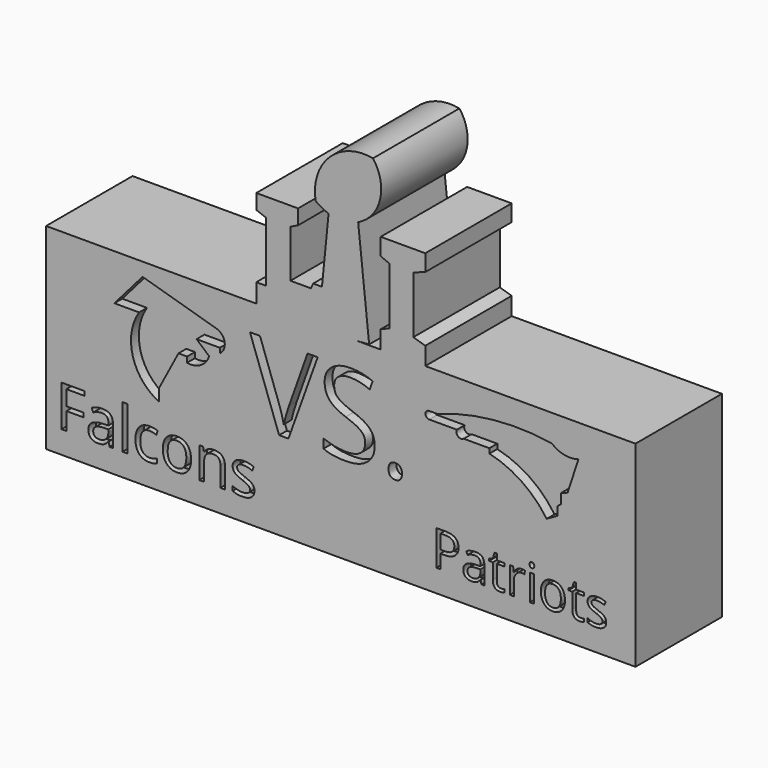
from build123d import *

# Parameters (mm, degrees)
F1_DEPTH       = 27.94
F2_TEXT_SIZE   = 14.8749987905
F2_TEXT_SIZE_2 = 12.6875005662
F2_TEXT_SIZE_3 = 29.4177713774
F3_DEPTH       = 2.54


# Not quite as in the source:
# - Text() gives the source's letters only with a copy of the font that has no kerning and outlines rounded to 1/6400 em; it was checked with that copy


with BuildPart() as f1:
    # F0 (on Front) → F1 (new body)
    with BuildSketch(Plane.XZ):
        Polygon((-20.7396647019, 6.5645907312), (-75.0956647019, 6.5645907312), (-75.0956647019, -44.2354092688), (77.3043352981, -44.2354092688), (77.3043352981, 6.5645907312), (22.9483352981, 6.5645907312), (11.4252582135, 6.5645907312), (5.2129668421, 6.5645907312), align=None)
        with BuildLine():
            Line((-20.7396647019, 11.4441978476), (-20.7396647019, 6.5645907312))
            Line((-20.7396647019, 6.5645907312), (5.2129668421, 6.5645907312))
            Line((5.2129668421, 6.5645907312), (3.6289432175, 32.9649871859))
            ThreePointArc((3.6289432175, 32.9649871859), (0.777301251, 32.6608543414), (-2.049780525, 33.1424842033))
            Line((-2.049780525, 33.1424842033), (-3.7631863539, 15.9227544818))
            Line((-3.7631863539, 15.9227544818), (-6.0277319506, 15.9227544818))
            Line((-6.0277319506, 15.9227544818), (-6.6274235949, 14.6377006922))
            Line((-6.6274235949, 14.6377006922), (-11.9156263826, 14.6377006922))
            Line((-11.9156263826, 14.6377006922), (-11.9156263826, 26.9505194119))
            Line((-11.9156263826, 26.9505194119), (-9.9452095164, 27.8928911975))
            Line((-9.9452095164, 27.8928911975), (-9.9452095164, 31.7480562917))
            Line((-9.9452095164, 31.7480562917), (-20.7396647019, 31.7480562917))
            Line((-20.7396647019, 31.7480562917), (-20.7396647019, 27.8928911975))
            Line((-20.7396647019, 27.8928911975), (-18.2552276237, 26.9505194119))
            Line((-18.2552276237, 26.9505194119), (-18.2552276237, 11.4441978476))
            Line((-18.2552276237, 11.4441978476), (-20.7396647019, 11.4441978476))
        make_face()
        with BuildLine():
            Line((3.6289432175, 32.9649871859), (5.2129668421, 6.5645907312))
            Line((5.2129668421, 6.5645907312), (8.4404846862, 6.758241782))
            Line((8.4404846862, 6.758241782), (5.5982306723, 33.6702211093))
            ThreePointArc((5.5982306723, 33.6702211093), (4.6312572936, 33.26826166), (3.6289432175, 32.9649871859))
        make_face()
        Polygon((11.4252582135, 11.1887202485), (11.4252582135, 6.5645907312), (22.9483352981, 6.5645907312), (22.9483352981, 11.1887202485), (19.8673630075, 12.1255040675), (19.8673630075, 26.8694617361), (22.9483352981, 27.9540222956), (22.9483352981, 32.2345261348), (11.4252582135, 32.2345261348), (11.4252582135, 27.8206810862), (13.6844111549, 26.8694617361), (13.6844111549, 12.1255040675), align=None)
        with BuildLine():
            ThreePointArc((-2.049780525, 33.1424842033), (0.777301251, 32.6608543414), (3.6289432175, 32.9649871859))
            ThreePointArc((3.6289432175, 32.9649871859), (4.6312572936, 33.26826166), (5.5982306723, 33.6702211093))
            ThreePointArc((5.5982306723, 33.6702211093), (11.2702064802, 40.6482895305), (9.43088028, 49.4506544164))
            ThreePointArc((9.43088028, 49.4506544164), (-1.7919494105, 46.0737788777), (-5.3994817717, 34.922953575))
            ThreePointArc((-5.3994817717, 34.922953575), (-3.8060075962, 33.8796206145), (-2.049780525, 33.1424842033))
        make_face()
    extrude(amount=F1_DEPTH)

    # F2 (on face) → F3 (cut)
    with BuildSketch(Plane.XZ.offset(27.94)):
        with BuildLine():
            Line((-57.4300996959, -5.2845505534), (-51.0407872498, -5.2845505534))
            ThreePointArc((-51.0407872498, -5.2845505534), (-52.6724909786, -15.8235590914), (-45.8401814103, -24.0121306388))
            Line((-45.8401814103, -24.0121306388), (-45.8401814103, -20.7377706656))
            Line((-45.8401814103, -20.7377706656), (-40.8624634147, -11.3023910208))
            Line((-40.8624634147, -11.3023910208), (-38.6336296797, -11.3023910208))
            Line((-38.6336296797, -11.3023910208), (-38.6336296797, -12.7139836086))
            ThreePointArc((-38.6336296797, -12.7139836086), (-35.1501450384, -12.1175824753), (-32.9300854222, -9.3677288686))
            Line((-32.9300854222, -9.3677288686), (-36.1819192767, -6.5475543497))
            Line((-36.1819192767, -6.5475543497), (-30.164077878, -6.5475543497))
            Line((-30.164077878, -6.5475543497), (-30.164077878, -7.810558146))
            ThreePointArc((-30.164077878, -7.810558146), (-28.9298311029, -4.8559593753), (-31.0556106269, -2.4613653777))
            Line((-31.0556106269, -2.4613653777), (-50.1492545009, 3.1107096465))
            Line((-50.1492545009, 3.1107096465), (-57.4300996959, -5.2845505534))
        make_face()
        with BuildLine():
            Line((25.9901545942, -3.3205924092), (23.9691324532, -3.3205924092))
            ThreePointArc((23.9691324532, -3.3205924092), (22.9947119951, -4.2950128673), (23.9691324532, -5.2694333253))
            Line((23.9691324532, -5.2694333253), (31.1099886894, -5.2694333253))
            ThreePointArc((31.1099886894, -5.2694333253), (31.4155848558, -6.7063022104), (32.8838806599, -6.7520038692))
            Line((32.8838806599, -6.7520038692), (39.5359098911, -6.7520038692))
            Line((39.5359098911, -6.7520038692), (39.5359098911, -7.9800849317))
            ThreePointArc((39.5359098911, -7.9800849317), (47.8722252158, -11.61639135), (54.341096431, -18.0094018115))
            Line((54.341096431, -18.0094018115), (57.1915879846, -16.3833805827))
            Line((57.1915879846, -16.3833805827), (57.1915879846, -14.1751709862))
            Line((57.1915879846, -14.1751709862), (58.0271296203, -13.5186761154))
            Line((58.0271296203, -13.5186761154), (58.0271296203, -10.9523785768))
            Line((58.0271296203, -10.9523785768), (59.7578845918, -10.2958827747))
            Line((59.7578845918, -10.2958827747), (62.5523142517, -1.7819450704))
            ThreePointArc((62.5523142517, -1.7819450704), (58.9290224546, -1.9857674916), (55.6690357625, -0.3913165538))
            ThreePointArc((55.6690357625, -0.3913165538), (40.6429760443, 0.0348360683), (25.9901545942, -3.3205924092))
        make_face()
        with Locations((-72.5345332175, -38.4005177766)):
            Text('Falcons', F2_TEXT_SIZE, font='Open Sans', text_align=(TextAlign.LEFT, TextAlign.BOTTOM))
        with Locations((24.5656706393, -38.4204499424)):
            Text('Patriots', F2_TEXT_SIZE_2, font='Open Sans', text_align=(TextAlign.LEFT, TextAlign.BOTTOM))
        with Locations((-22.374120889, -21.4705977848)):
            Text('VS.', F2_TEXT_SIZE_3, font='Open Sans', text_align=(TextAlign.LEFT, TextAlign.BOTTOM))
    extrude(amount=-F3_DEPTH, mode=Mode.SUBTRACT)


solid = f1.part
